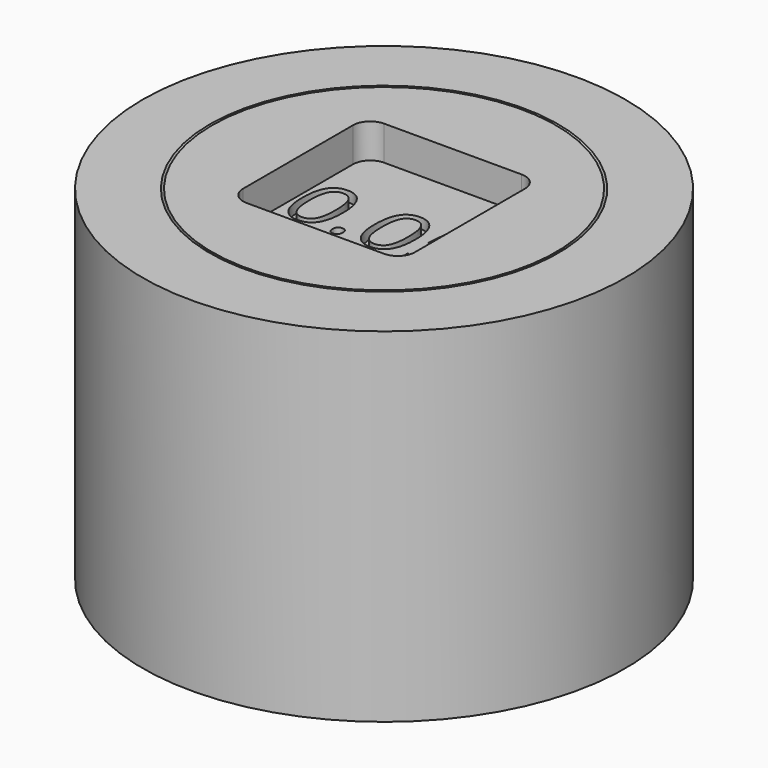
from build123d import *

# Parameters (mm, degrees)
F4_DEPTH     = 1
F5_TEXT_SIZE = 2.514339593
F6_DEPTH     = 1.3


# Not quite as in the source:
# - Text() gives the source's letters only with a copy of the font that has no kerning and outlines rounded to 1/6400 em; it was checked with that copy


with BuildPart() as f1:
    # F0 (on Front) → F1 (revolve)
    with BuildSketch(Plane.XZ):
        with BuildLine():
            Line((-5, 0), (0, 0))
            Line((0, 0), (0, 10))
            Line((0, 10), (-5, 10))
            Line((-5, 10), (-2.7928932188, 7.7928932188))
            ThreePointArc((-2.7928932188, 7.7928932188), (-2.5761204675, 7.46846987), (-2.5, 7.0857864376))
            Line((-2.5, 7.0857864376), (-2.5, 2.9142135624))
            ThreePointArc((-2.5, 2.9142135624), (-2.5761204675, 2.53153013), (-2.7928932188, 2.2071067812))
            Line((-2.7928932188, 2.2071067812), (-5, 0))
        make_face()
    revolve(axis=Axis((0, 0, 5), (0, 0, 1)))

    # F3 (on face) → F4 (cut)
    with BuildSketch(Plane.XY.offset(10)):
        with BuildLine():
            Line((2, 2.5), (-2, 2.5))
            ThreePointArc((-2, 2.5), (-2.3535533906, 2.3535533906), (-2.5, 2))
            Line((-2.5, 2), (-2.5, -2))
            ThreePointArc((-2.5, -2), (-2.3535533906, -2.3535533906), (-2, -2.5))
            Line((-2, -2.5), (2, -2.5))
            ThreePointArc((2, -2.5), (2.3535533906, -2.3535533906), (2.5, -2))
            Line((2.5, -2), (2.5, 2))
            ThreePointArc((2.5, 2), (2.3535533906, 2.3535533906), (2, 2.5))
        make_face()
    extrude(amount=-F4_DEPTH, mode=Mode.SUBTRACT)

    # F5 (on offset) → F6 (cut)
    with BuildSketch(Plane.XY.offset(10)):
        with Locations((-2.5, -0.9051622535)):
            Text('0.05', F5_TEXT_SIZE, font='Open Sans', text_align=(TextAlign.LEFT, TextAlign.BOTTOM))
    extrude(amount=-F6_DEPTH, mode=Mode.SUBTRACT)


with BuildPart() as f1b:
    # F0 (on Front) → F1, piece 2 (revolve)
    with BuildSketch(Plane.XZ):
        with BuildLine():
            Line((-7.0207106781, 10), (-7.0207106781, 0))
            Line((-7.0207106781, 0), (-5.0707106781, 0))
            Line((-5.0707106781, 0), (-2.8428932188, 2.2278174593))
            ThreePointArc((-2.8428932188, 2.2278174593), (-2.6261204675, 2.5522408081), (-2.55, 2.9349242405))
            Line((-2.55, 2.9349242405), (-2.55, 7.0650757595))
            ThreePointArc((-2.55, 7.0650757595), (-2.6261204675, 7.4477591919), (-2.8428932188, 7.7721825407))
            Line((-2.8428932188, 7.7721825407), (-5.0707106781, 10))
            Line((-5.0707106781, 10), (-7.0207106781, 10))
        make_face()
    revolve(axis=Axis((0, 0, 5), (0, 0, 1)))


solid = Compound([f1.part, f1b.part])
